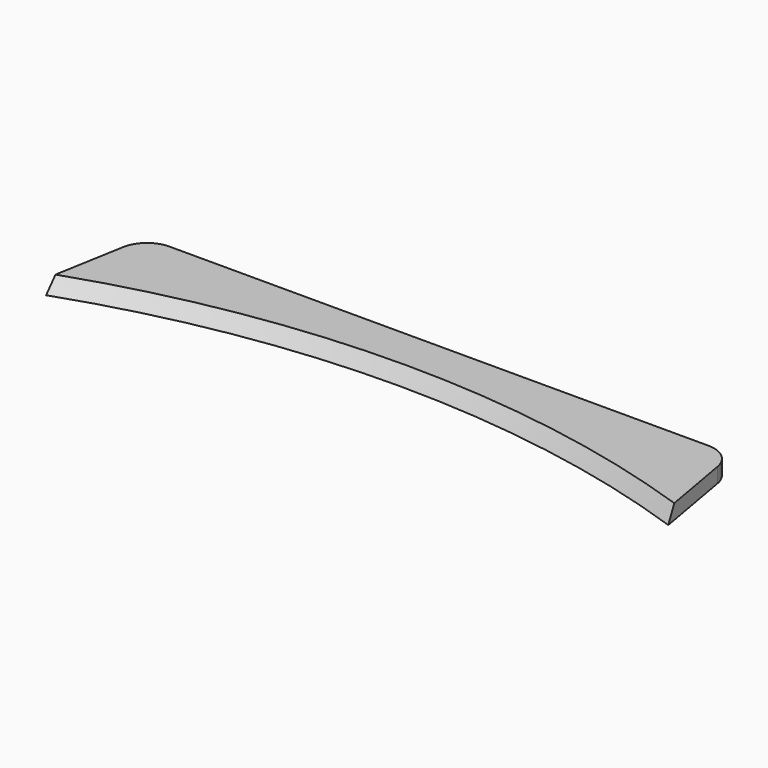
from build123d import *

# Parameters (mm, degrees)
F1_DEPTH = 15.875
F2_SIZE2 = 9.165426
F2_SIZE  = 15.87499


# Not quite as in the source:
# - a fillet or chamfer is up to 0.001 mm smaller than in the source, because OpenCascade refuses the exact size


with BuildPart() as f1:
    # F0 (on Top) → F1 (new body)
    with BuildSketch(Plane.XY):
        with BuildLine():
            ThreePointArc((-333.375, 0), (0, 56.2515384878), (333.375, 0))
            Line((333.375, 0), (318.4555045755, 84.6126631589))
            ThreePointArc((318.4555045755, 84.6126631589), (308.1393220024, 102.4808155156), (288.7512407253, 109.5375))
            Line((288.7512407253, 109.5375), (-288.7512407253, 109.5375))
            ThreePointArc((-288.7512407253, 109.5375), (-308.1393220024, 102.4808155156), (-318.4555045755, 84.6126631589))
            Line((-318.4555045755, 84.6126631589), (-333.375, 0))
        make_face()
    extrude(amount=F1_DEPTH)

    # F2 (size 15.875 and 9.1654355234 in the source; OpenCascade refuses exactly that, so slightly less here)
    f2_edges = [f1.edges().sort_by_distance(p)[0] for p in [
        (0, 56.251538, 15.875),
    ]]
    f2_side = f1.faces().sort_by_distance((0, 56.251538, 7.9375))[0]
    chamfer(f2_edges, length=F2_SIZE, length2=F2_SIZE2, reference=f2_side)


solid = f1.part
